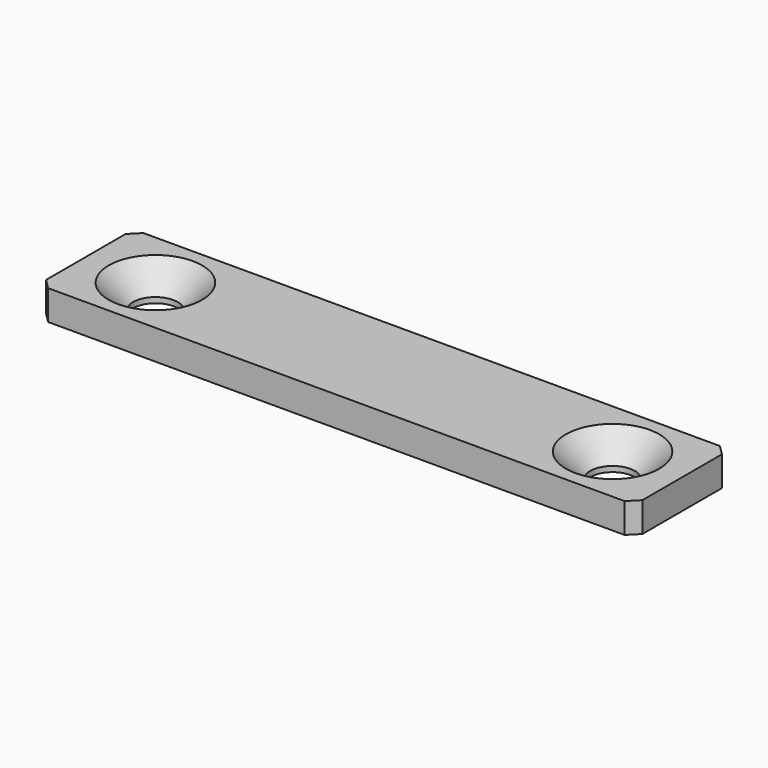
from build123d import *

# Parameters (mm, degrees)
F0_W           = 60
F0_H           = 12
F1_DEPTH       = 3
F3_D           = 4.5
F3_DEPTH       = 3.4
F3_CSINK_D     = 9.4
F3_CSINK_ANGLE = 90
F3_TIP         = 1.3519363928
F4_SIZE        = 1


with BuildPart() as f1:
    # F0 (on Top) → F1 (new body)
    with BuildSketch(Plane.XY):
        Rectangle(F0_W, F0_H)
    extrude(amount=F1_DEPTH)

    # F3
    with Locations(Plane.XY.offset(3)):
        with Locations((-23, 0), (23, 0)):
            CounterSinkHole(F3_D / 2, F3_CSINK_D / 2, depth=F3_DEPTH, counter_sink_angle=F3_CSINK_ANGLE)
            with Locations((0, 0, -(F3_DEPTH + F3_TIP / 2))):  # 118° drill point
                Cone(0, F3_D / 2, F3_TIP, mode=Mode.SUBTRACT)

    # F4
    f4_edges = [f1.edges().sort_by_distance(p)[0] for p in [
        (30, 6, 1.5),
        (30, -6, 1.5),
        (-30, -6, 1.5),
        (-30, 6, 1.5),
    ]]
    chamfer(f4_edges, length=F4_SIZE)


solid = f1.part
